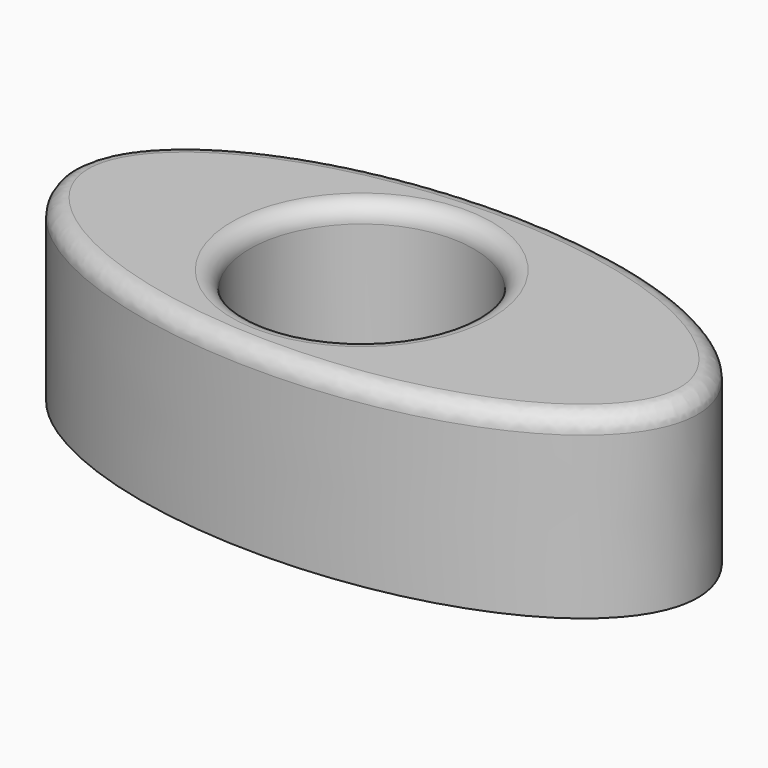
from build123d import *

# Parameters (mm, degrees)
F1_DEPTH = 25.4
F2_R     = 2.54
F3_R     = 2.54


# Not quite as in the source:
# - a feature names something its author has since deleted; it is built from what else it names


with BuildPart() as f1:
    # F0 (on Top) → F1 (new body)
    with BuildSketch(Plane.XY):
        with BuildLine():
            add(Edge.make_bspline(
                [(47.6249848312, -0.0183610014), (47.6249848312, 22.1974603925), (3.1933458341, 22.2066371025), (-41.2382931629, 22.2158138126), (-41.275, 0)],
                knots=[0, 0, 0, 1.5703832559, 1.5703832559, 3.1407665117, 3.1407665117, 3.1407665117], degree=2, weights=[1, 0.7072528087, 1, 0.7072528087, 1]))
            add(Edge.make_bspline(
                [(-41.275, 0), (-41.3117371747, -22.2341748108), (3.1566238283, -22.2433591053), (47.6249848312, -22.2525433997), (47.6249848312, -0.0183610014)],
                knots=[3.1407665117, 3.1407665117, 3.1407665117, 4.7119759094, 4.7119759094, 6.2831853072, 6.2831853072, 6.2831853072], degree=2, weights=[1, 0.7069607235, 1, 0.7069607235, 1]))
        make_face()
        with BuildLine():
            ThreePointArc((-15.875, 0), (0, 15.875), (15.875, 0))
            ThreePointArc((15.875, 0), (0, -15.875), (-15.875, 0))
        make_face(mode=Mode.SUBTRACT)
    extrude(amount=F1_DEPTH)

    # F2
    f2_edges = [f1.edges().sort_by_distance(p)[0] for p in [
        (3.165804, -22.243361, 25.4),
    ]]
    fillet(f2_edges, radius=F2_R)

    # F3
    f3_edges = [f1.edges().sort_by_distance(p)[0] for p in [
        (-15.875, 0, 25.4),
    ]]
    fillet(f3_edges, radius=F3_R)


solid = f1.part
